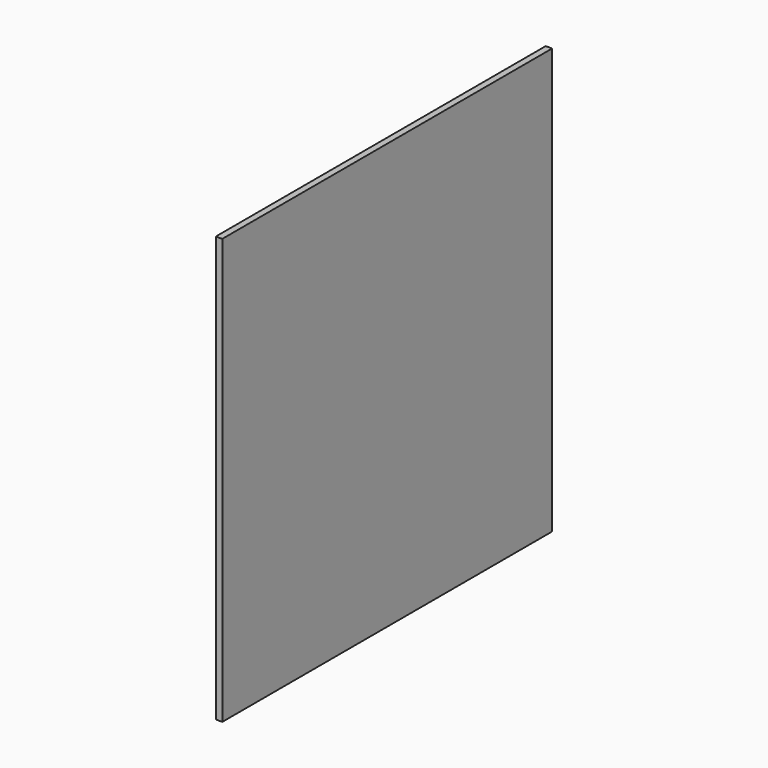
from build123d import *

# Parameters (mm, degrees)
F0_W     = 812.8
F0_H     = 838.2
F1_DEPTH = 12.7


# Not quite as in the source:
# - a length typed as a fraction of an inch, garbled in the dataset ("3 / 203.2 mm" for 3/8 in), is restored


with BuildPart() as f1:
    # F0 (on Right) → F1 (new body)
    with BuildSketch(Plane.YZ):
        with Locations((2.8780587018, 80.8559241794)):
            Rectangle(F0_W, F0_H)
    extrude(amount=F1_DEPTH)


solid = f1.part
